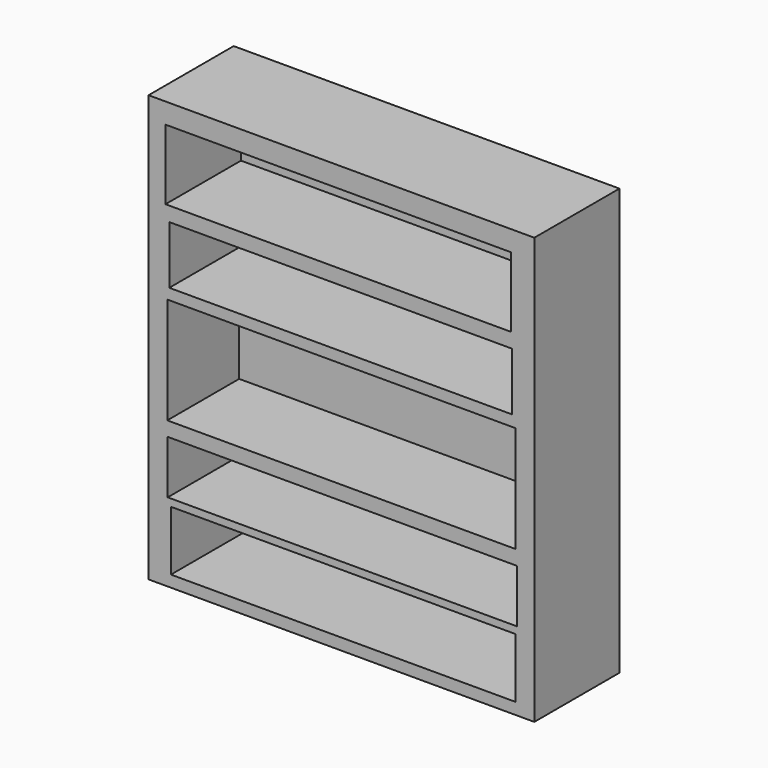
from build123d import *

# Parameters (mm, degrees)
F0_W      = 138.1484791636
F0_H      = 52.3216351867
F1_DEPTH  = 38.1
F2_W      = 124.6868036687
F2_H      = 5.9200678952
F3_DEPTH  = 38.1
F4_W      = 138.1484791636
F4_H      = 38.1
F5_DEPTH  = 2.54
F6_W      = 138.1484791636
F6_H      = 38.1
F7_DEPTH  = 59.69
F8_W      = 122.7258816361
F8_H      = 20.7270383835
F12_DEPTH = 33.782
F9_W      = 123.8167844713
F9_H      = 25.0906273723
F13_DEPTH = 33.782
F10_W     = 125.1115500927
F10_H     = 19.0701205283
F14_DEPTH = 33.782
F11_W     = 123.3779042959
F11_H     = 21.381651517
F15_DEPTH = 33.782


# Not quite as in the source:
# - a feature names something its author has since deleted; it is built from what else it names


with BuildPart() as f1:
    # F0 (on Front) → F1 (new body)
    with BuildSketch(Plane.XZ):
        with Locations((0.4136152565, 26.1608175933)):
            Rectangle(F0_W, F0_H)
    extrude(amount=F1_DEPTH)

    # F2 (on face) → F3 (join)
    with BuildSketch(Plane.XY.offset(52.3216351867)):
        Polygon((-61.9600676, 0), (-68.6606243253, 0), (-68.6606243253, -38.1), (-61.9600676, -38.1), (-61.9600676, -5.9200678952), align=None)
        with Locations((0.3833342344, -2.9600339476)):
            Rectangle(F2_W, F2_H)
        Polygon((69.4878548384, 0), (62.7267360687, 0), (62.7267360687, -5.9200678952), (62.7267360687, -38.1), (69.4878548384, -38.1), align=None)
    extrude(amount=F3_DEPTH)

    # F4 (on face) → F5 (join)
    with BuildSketch(Plane.XY.offset(90.4216351867)):
        with Locations((0.4136152565, -19.05)):
            Rectangle(F4_W, F4_H)
    extrude(amount=F5_DEPTH)

    # F6 (on face) → F7 (join)
    with BuildSketch(Plane.XY.offset(92.9616351867)):
        with Locations((0.4136152565, -19.05)):
            Rectangle(F6_W, F6_H)
    extrude(amount=F7_DEPTH)

    # F8 (on face) → F12 (cut)
    with BuildSketch(Plane.XZ.offset(38.1)):
        with Locations((0.1238100231, 104.7143563628)):
            Rectangle(F8_W, F8_H)
    extrude(amount=-F12_DEPTH, mode=Mode.SUBTRACT)

    # F9 (on face) → F13 (cut)
    with BuildSketch(Plane.XZ.offset(38.1)):
        with Locations((-0.694366172, 132.8049488366)):
            Rectangle(F9_W, F9_H)
    extrude(amount=-F13_DEPTH, mode=Mode.SUBTRACT)

    # F10 (on face) → F14 (cut)
    with BuildSketch(Plane.XZ.offset(38.1)):
        with Locations((0.7500052452, 37.6429138705)):
            Rectangle(F10_W, F10_H)
    extrude(amount=-F14_DEPTH, mode=Mode.SUBTRACT)

    # F11 (on face) → F15 (cut)
    with BuildSketch(Plane.XZ.offset(38.1)):
        with Locations((1.0389462113, 14.81655729)):
            Rectangle(F11_W, F11_H)
    extrude(amount=-F15_DEPTH, mode=Mode.SUBTRACT)


solid = f1.part
